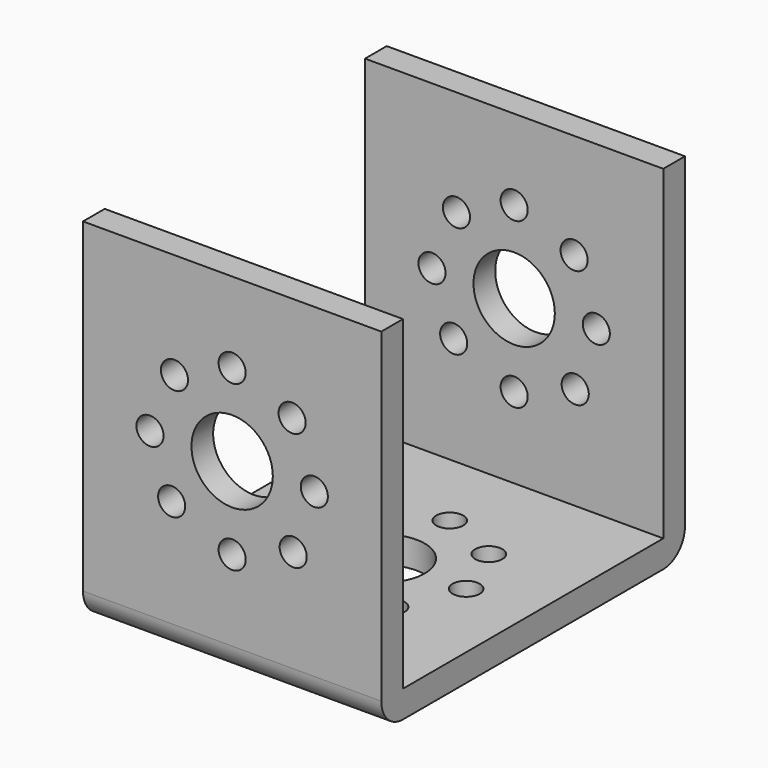
from build123d import *

# Parameters (mm, degrees)
F0_W     = 27.94
F0_H     = 33.02
F1_DEPTH = 17.78
F2_T     = -2.54
F3_R     = 2.54
F5_D     = 7.62
F7_D     = 7.62
F9_D     = 2.54
F11_D    = 2.54


# Not quite as in the source:
# - a feature names something its author has since deleted; it is built from what else it names


with BuildPart() as f1:
    # F0 (on Front) → F1 (new body, symmetric)
    with BuildSketch(Plane.XZ):
        Rectangle(F0_W, F0_H)
    extrude(amount=F1_DEPTH, both=True)

    # F2
    f2_openings = [f1.faces().sort_by_distance(p)[0] for p in [
        (0, 0, 16.51),
        (-13.97, 0, 0),
        (13.97, 0, 0),
    ]]
    offset(amount=F2_T, openings=f2_openings)

    # F3
    f3_edges = [f1.edges().sort_by_distance(p)[0] for p in [
        (0, 17.78, -16.51),
        (0, -17.78, -16.51),
    ]]
    fillet(f3_edges, radius=F3_R)

    # F5 (through all)
    with Locations(Plane.XY.offset(-13.97)):
        with Locations((0, 0)):
            Hole(F5_D / 2)

    # F7 (through all)
    with Locations(Plane(origin=(0, 17.78, 0), x_dir=(-1, 0, 0), z_dir=(0, 1, 0))):
        with Locations((0, 1.2737165671)):
            Hole(F7_D / 2)

    # F9 (through all)
    with Locations(Plane.XZ.offset(17.78)):
        with Locations((-5.4043098353, 6.6219973378), (0, 8.9699165671), (5.6151403114, 6.673975382), (7.6956628408, 1.2737165671), (5.7190973312, -4.3454747647), (0, -6.4224834329), (-5.6642023847, -3.8776681758), (-7.6962, 1.2737165671)):
            Hole(F9_D / 2)

    # F11 (through all)
    with Locations(Plane(origin=(0, 0, -16.51), x_dir=(1, 0, 0), z_dir=(0, 0, -1))):
        with Locations((-5.1595509827, 5.7105628529), (0, 7.6962), (5.2015446278, 5.6723388408), (7.6962, 0), (-5.7603712318, -5.1038826115), (-7.6962, 0), (0, -7.6962), (5.5570431587, -5.3245437149)):
            Hole(F11_D / 2)


solid = f1.part
